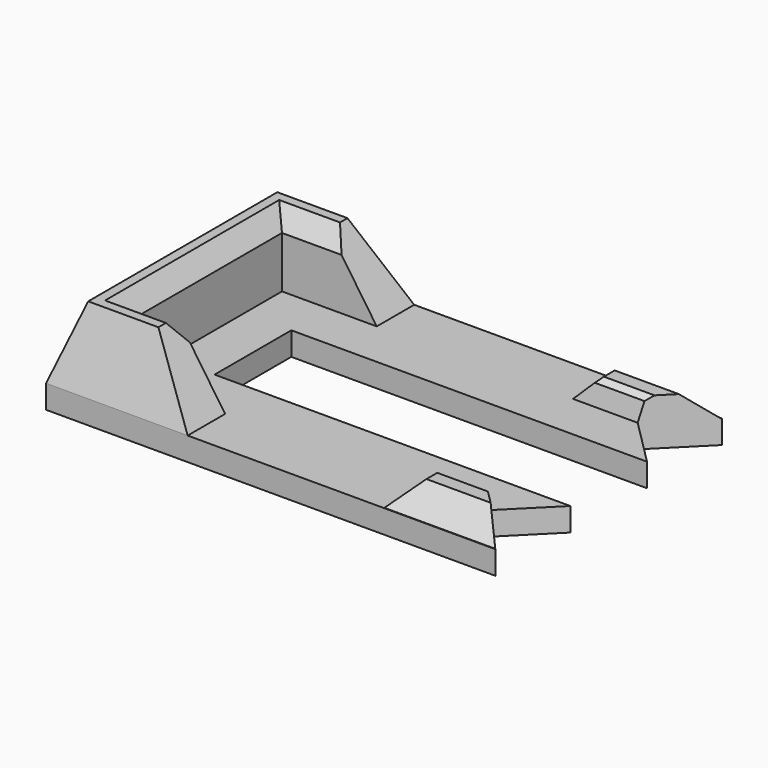
from build123d import *

# Parameters (mm, degrees)
F0_W           = 172
F0_H           = 60.5
F4_DEPTH       = 5
F6_SIZE2       = 4
F6_SIZE        = 3
F9_DEPTH       = 5
F10_SIZE       = 4.99999
F11_SIZE2      = 0.99999
F11_SIZE       = 4.99999
F12_SIZE       = 1
F14_W          = 132
F14_H          = 20.5
F15_DEPTH      = 12.5
F17_DEPTH      = 25
F17_DEPTH_BACK = 25


# Not quite as in the source:
# - a fillet or chamfer is up to 0.001 mm smaller than in the source, because OpenCascade refuses the exact size


with BuildPart() as f4:
    # F0 (on Top) → F4 (new body)
    with BuildSketch(Plane.XY):
        Rectangle(F0_W, F0_H)
    extrude(amount=-F4_DEPTH)

    # F3 (on Top) → F5 section 0
    with BuildSketch(Plane.XY):
        Polygon((-86, 0), (-86, -30.25), (-55.75, -30.25), (-55.75, -20.25), (-76, -20.25), (-76, 0), align=None)
    # F2 (on offset) → F5 section 1
    with BuildSketch(Plane.XY.offset(15)):
        Polygon((-76, -20.25), (-76, 0), (-81, 0), (-81, -25.25), (-66, -25.25), (-66, -20.25), align=None)
    loft()

    # F6
    f6_edges = [f4.edges().sort_by_distance(p)[0] for p in [
        (-76, -10.125, 15),
        (-71, -20.25, 15),
    ]]
    chamfer(f6_edges, length=F6_SIZE, length2=F6_SIZE2)

    # F7: F4 across plane


with BuildPart() as f4_1:
    add(f4.part)
    add(f4.part.mirror(Plane.YZ))

    # F8 (on face) → F9 (join)
    with BuildSketch(Plane.XY):
        Polygon((13.8189587742, -20.25), (0, -20.25), (-13.8189587742, -20.25), (-13.8189587742, -30.1344580948), (0, -30.1344580948), (13.8189587742, -30.1344580948), align=None)
    extrude(amount=F9_DEPTH)

    # F10 (size 5 in the source; OpenCascade refuses exactly that, so slightly less here)
    f10_edges = [f4_1.edges().sort_by_distance(p)[0] for p in [
        (13.818959, -25.192229, 5),
        (0, -30.134458, 5),
        (-13.818959, -25.192229, 5),
    ]]
    chamfer(f10_edges, length=F10_SIZE)

    # F11 (size 5 and 1 in the source; OpenCascade refuses exactly that, so slightly less here)
    f11_edges = [f4_1.edges().sort_by_distance(p)[0] for p in [
        (0, -20.25, 5),
    ]]
    f11_side = f4_1.faces().sort_by_distance((0, -20.25, 2.315943))[0]
    chamfer(f11_edges, length=F11_SIZE, length2=F11_SIZE2, reference=f11_side)

    # F12
    f12_edges = [f4_1.edges().sort_by_distance(p)[0] for p in [
        (0, -21.24999, 5),
    ]]
    chamfer(f12_edges, length=F12_SIZE)

    # F13: F4 across plane


with BuildPart() as f4_2:
    add(f4_1.part)
    add(f4_1.part.mirror(Plane.XZ))

    # F14 (on Top) → F15 (cut, symmetric)
    with BuildSketch(Plane.XY):
        Rectangle(F14_W, F14_H)
    extrude(amount=F15_DEPTH, both=True, mode=Mode.SUBTRACT)


with BuildPart() as f17:
    # F16 (on Top) → F17 (new body, two sides)
    with BuildSketch(Plane.XY) as f17_sk:
        Polygon((23.7979591321, 44.0479591321), (0, 20.25), (18.644013716, 1.605986284), (18.644013716, -1.605986284), (0, -20.25), (26.894013716, -47.144013716), (91.0670285058, -47.144013716), (91.0670285058, 44.0479591321), align=None)
    extrude(amount=F17_DEPTH)
    extrude(f17_sk.sketch, amount=-F17_DEPTH_BACK)


with BuildPart() as f4_3:
    add(f4_2.part)

    # F18: cut F17
    add(f17.part, mode=Mode.SUBTRACT)


solid = f4_3.part
